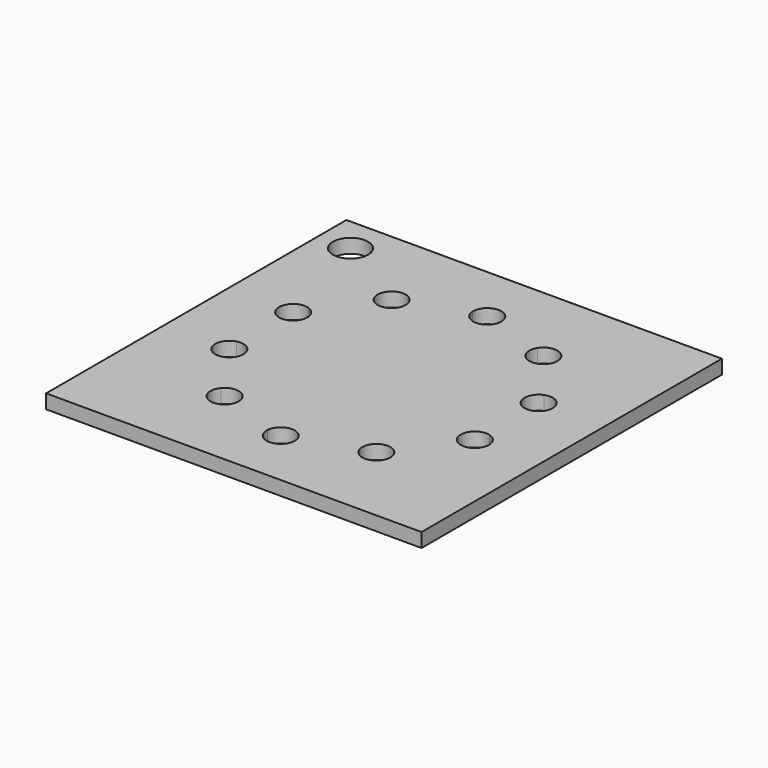
from build123d import *

# Parameters (mm, degrees)
F0_W     = 80
F0_H     = 80
F1_DEPTH = 3
F3_DEPTH = 25
F4_R     = 3.75
F5_DEPTH = 25


with BuildPart() as f1:
    # F0 (on Top) → F1 (new body)
    with BuildSketch(Plane.XY):
        Rectangle(F0_W, F0_H)
    extrude(amount=F1_DEPTH)

    # F2 (on face) → F3 (cut)
    with BuildSketch(Plane.XY.offset(3)):
        with BuildLine():
            ThreePointArc((25.0727558965, 11.2963229308), (23.3008846492, 7.5709163622), (26.9240976399, 5.5984789253))
            ThreePointArc((26.9240976399, 5.5984789253), (26.1540541981, 8.4979673453), (25.0727558965, 11.2963229308))
        make_face()
        with BuildLine():
            ThreePointArc((25.0727558965, 11.2963229308), (26.1540541981, 8.4979673453), (26.9240976399, 5.5984789253))
            ThreePointArc((26.9240976399, 5.5984789253), (28.5320922892, 6.669051044), (29.1540541981, 8.4979673453))
            ThreePointArc((29.1540541981, 8.4979673453), (27.8505366022, 10.9722242949), (25.0727558965, 11.2963229308))
        make_face()
        with BuildLine():
            ThreePointArc((29.1540541981, -8.4979673453), (28.5320922892, -6.669051044), (26.9240976399, -5.5984789253))
            ThreePointArc((26.9240976399, -5.5984789253), (26.1540541981, -8.4979673453), (25.0727558965, -11.2963229308))
            ThreePointArc((25.0727558965, -11.2963229308), (27.8505366022, -10.9722242949), (29.1540541981, -8.4979673453))
        make_face()
        with BuildLine():
            ThreePointArc((25.0727558965, -11.2963229308), (26.1540541981, -8.4979673453), (26.9240976399, -5.5984789253))
            ThreePointArc((26.9240976399, -5.5984789253), (23.3008846492, -7.5709163622), (25.0727558965, -11.2963229308))
        make_face()
        with BuildLine():
            ThreePointArc((13.6444735922, 23.8763133752), (14.4007386812, 19.8209163622), (18.4913492013, 20.3548521172))
            ThreePointArc((18.4913492013, 20.3548521172), (16.164094438, 22.2479673453), (13.6444735922, 23.8763133752))
        make_face()
        with BuildLine():
            ThreePointArc((13.6444735922, 23.8763133752), (16.164094438, 22.2479673453), (18.4913492013, 20.3548521172))
            ThreePointArc((18.4913492013, 20.3548521172), (18.990909279, 21.2434187626), (19.164094438, 22.2479673453))
            ThreePointArc((19.164094438, 22.2479673453), (17.0129576374, 25.1253674337), (13.6444735922, 23.8763133752))
        make_face()
        with BuildLine():
            ThreePointArc((19.164094438, -22.2479673453), (18.990909279, -21.2434187626), (18.4913492013, -20.3548521172))
            ThreePointArc((18.4913492013, -20.3548521172), (16.164094438, -22.2479673453), (13.6444735922, -23.8763133752))
            ThreePointArc((13.6444735922, -23.8763133752), (17.0129576374, -25.1253674337), (19.164094438, -22.2479673453))
        make_face()
        with BuildLine():
            ThreePointArc((13.6444735922, -23.8763133752), (16.164094438, -22.2479673453), (18.4913492013, -20.3548521172))
            ThreePointArc((18.4913492013, -20.3548521172), (14.4007386812, -19.8209163622), (13.6444735922, -23.8763133752))
        make_face()
        with BuildLine():
            ThreePointArc((-2.9955338657, 27.3363636364), (0, 24.5), (2.9955338657, 27.3363636364))
            ThreePointArc((2.9955338657, 27.3363636364), (0, 27.5), (-2.9955338657, 27.3363636364))
        make_face()
        with BuildLine():
            ThreePointArc((-2.9955338657, 27.3363636364), (0, 27.5), (2.9955338657, 27.3363636364))
            ThreePointArc((2.9955338657, 27.3363636364), (2.9988832586, 27.4181513503), (3, 27.5))
            ThreePointArc((3, 27.5), (-0.0818486497, 30.4988832586), (-2.9955338657, 27.3363636364))
        make_face()
        with BuildLine():
            ThreePointArc((3, -27.5), (2.9988832586, -27.4181513503), (2.9955338657, -27.3363636364))
            ThreePointArc((2.9955338657, -27.3363636364), (0, -27.5), (-2.9955338657, -27.3363636364))
            ThreePointArc((-2.9955338657, -27.3363636364), (-0.0818486497, -30.4988832586), (3, -27.5))
        make_face()
        with BuildLine():
            ThreePointArc((-2.9955338657, -27.3363636364), (0, -27.5), (2.9955338657, -27.3363636364))
            ThreePointArc((2.9955338657, -27.3363636364), (0, -24.5), (-2.9955338657, -27.3363636364))
        make_face()
        with BuildLine():
            ThreePointArc((-13.164094438, 22.2479673453), (-13.2866943496, 23.0968305447), (-13.6444735922, 23.8763133752))
            ThreePointArc((-13.6444735922, 23.8763133752), (-16.164094438, 22.2479673453), (-18.4913492013, 20.3548521172))
            ThreePointArc((-18.4913492013, 20.3548521172), (-15.1595458553, 19.4211525044), (-13.164094438, 22.2479673453))
        make_face()
        with BuildLine():
            ThreePointArc((-18.4913492013, 20.3548521172), (-16.164094438, 22.2479673453), (-13.6444735922, 23.8763133752))
            ThreePointArc((-13.6444735922, 23.8763133752), (-17.9274501949, 24.6750183284), (-18.4913492013, 20.3548521172))
        make_face()
        with BuildLine():
            ThreePointArc((-18.4913492013, -20.3548521172), (-17.9274501949, -24.6750183284), (-13.6444735922, -23.8763133752))
            ThreePointArc((-13.6444735922, -23.8763133752), (-16.164094438, -22.2479673453), (-18.4913492013, -20.3548521172))
        make_face()
        with BuildLine():
            ThreePointArc((-18.4913492013, -20.3548521172), (-16.164094438, -22.2479673453), (-13.6444735922, -23.8763133752))
            ThreePointArc((-13.6444735922, -23.8763133752), (-13.2866943496, -23.0968305447), (-13.164094438, -22.2479673453))
            ThreePointArc((-13.164094438, -22.2479673453), (-15.1595458553, -19.4211525044), (-18.4913492013, -20.3548521172))
        make_face()
        with BuildLine():
            ThreePointArc((-23.1540541981, 8.4979673453), (-23.6797972485, 10.1944497494), (-25.0727558965, 11.2963229308))
            ThreePointArc((-25.0727558965, 11.2963229308), (-26.1540541981, 8.4979673453), (-26.9240976399, 5.5984789253))
            ThreePointArc((-26.9240976399, 5.5984789253), (-24.3251378968, 6.1199292542), (-23.1540541981, 8.4979673453))
        make_face()
        with BuildLine():
            ThreePointArc((-26.9240976399, 5.5984789253), (-26.1540541981, 8.4979673453), (-25.0727558965, 11.2963229308))
            ThreePointArc((-25.0727558965, 11.2963229308), (-29.007223747, 9.4250183284), (-26.9240976399, 5.5984789253))
        make_face()
        with BuildLine():
            ThreePointArc((-26.9240976399, -5.5984789253), (-29.007223747, -9.4250183284), (-25.0727558965, -11.2963229308))
            ThreePointArc((-25.0727558965, -11.2963229308), (-26.1540541981, -8.4979673453), (-26.9240976399, -5.5984789253))
        make_face()
        with BuildLine():
            ThreePointArc((-26.9240976399, -5.5984789253), (-26.1540541981, -8.4979673453), (-25.0727558965, -11.2963229308))
            ThreePointArc((-25.0727558965, -11.2963229308), (-23.6797972485, -10.1944497494), (-23.1540541981, -8.4979673453))
            ThreePointArc((-23.1540541981, -8.4979673453), (-24.3251378968, -6.1199292542), (-26.9240976399, -5.5984789253))
        make_face()
    extrude(amount=-F3_DEPTH, mode=Mode.SUBTRACT)

    # F4 (on face) → F5 (cut)
    with BuildSketch(Plane.XY.offset(3)):
        with Locations((-33.1107974052, 32.4715934694)):
            Circle(F4_R)
    extrude(amount=-F5_DEPTH, mode=Mode.SUBTRACT)


solid = f1.part
